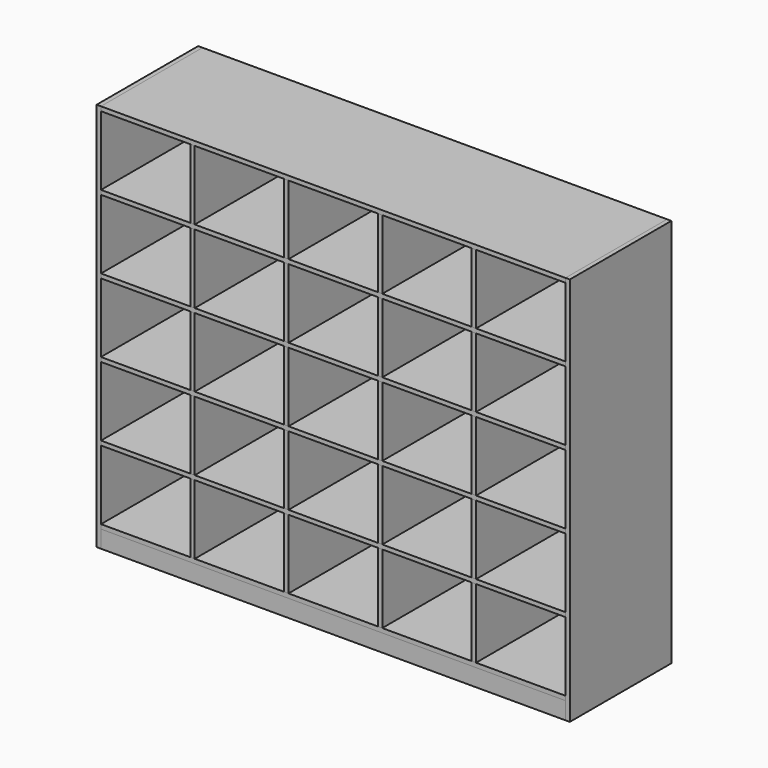
from build123d import *

# Parameters (mm, degrees)
F2_W      = 2044.7
F2_H      = 76.2
F6_DEPTH  = 19.05
F7_START  = -539.75
F7_DEPTH  = 19.05
F3_W      = 2044.7
F3_H      = 19.05
F8_DEPTH  = 558.8
F4_W      = 19.05
F4_H      = 1714.5000293255
F9_DEPTH  = 558.8
F5_W      = 19.05
F5_H      = 304.8000058651
F10_DEPTH = 558.8


# Not quite as in the source:
# - a variable given as a bare number and used for a length is read in inches; the dataset says mm whatever the document's units were


with BuildPart() as f6:
    # F2 (on Front) → F6 (new body)
    with BuildSketch(Plane.XZ):
        with Locations((0, 38.1)):
            Rectangle(F2_W, F2_H)
    extrude(amount=-F6_DEPTH)


with BuildPart() as f7:
    # F2 (on Front) → F7 (new body)
    with BuildSketch(Plane.XZ.offset(F7_START)):
        with Locations((0, 38.1)):
            Rectangle(F2_W, F2_H)
    extrude(amount=-F7_DEPTH)


with BuildPart() as f8:
    # F3 (on Front) → F8 (new body)
    with BuildSketch(Plane.XZ):
        with Locations((0, 85.725)):
            Rectangle(F3_W, F3_H)
    extrude(amount=-F8_DEPTH)


with BuildPart() as f8b:
    # F3 (on Front) → F8, piece 2 (new body)
    with BuildSketch(Plane.XZ):
        with Locations((0, 409.5750058651)):
            Rectangle(F3_W, F3_H)
    extrude(amount=-F8_DEPTH)


with BuildPart() as f8c:
    # F3 (on Front) → F8, piece 3 (new body)
    with BuildSketch(Plane.XZ):
        with Locations((0, 733.4250117302)):
            Rectangle(F3_W, F3_H)
    extrude(amount=-F8_DEPTH)


with BuildPart() as f8d:
    # F3 (on Front) → F8, piece 4 (new body)
    with BuildSketch(Plane.XZ):
        with Locations((0, 1057.2750175953)):
            Rectangle(F3_W, F3_H)
    extrude(amount=-F8_DEPTH)


with BuildPart() as f8e:
    # F3 (on Front) → F8, piece 5 (new body)
    with BuildSketch(Plane.XZ):
        with Locations((0, 1381.1250234604)):
            Rectangle(F3_W, F3_H)
    extrude(amount=-F8_DEPTH)


with BuildPart() as f8f:
    # F3 (on Front) → F8, piece 6 (new body)
    with BuildSketch(Plane.XZ):
        with Locations((0, 1704.9750293255)):
            Rectangle(F3_W, F3_H)
    extrude(amount=-F8_DEPTH)


with BuildPart() as f9:
    # F4 (on Front) → F9 (new body)
    with BuildSketch(Plane.XZ):
        with Locations((-1031.875, 857.2500146627)):
            Rectangle(F4_W, F4_H)
    extrude(amount=-F9_DEPTH)


with BuildPart() as f9b:
    # F4 (on Front) → F9, piece 2 (new body)
    with BuildSketch(Plane.XZ):
        with Locations((1031.875, 857.2500146627)):
            Rectangle(F4_W, F4_H)
    extrude(amount=-F9_DEPTH)


with BuildPart() as f10:
    # F5 (on Front) → F10 (new body)
    with BuildSketch(Plane.XZ):
        with Locations((-619.125, 247.6500029325)):
            Rectangle(F5_W, F5_H)
    extrude(amount=-F10_DEPTH)


with BuildPart() as f10b:
    # F5 (on Front) → F10, piece 2 (new body)
    with BuildSketch(Plane.XZ):
        with Locations((-619.125, 571.5000087976)):
            Rectangle(F5_W, F5_H)
    extrude(amount=-F10_DEPTH)


with BuildPart() as f10c:
    # F5 (on Front) → F10, piece 3 (new body)
    with BuildSketch(Plane.XZ):
        with Locations((-619.125, 895.3500146627)):
            Rectangle(F5_W, F5_H)
    extrude(amount=-F10_DEPTH)


with BuildPart() as f10d:
    # F5 (on Front) → F10, piece 4 (new body)
    with BuildSketch(Plane.XZ):
        with Locations((-619.125, 1219.2000205278)):
            Rectangle(F5_W, F5_H)
    extrude(amount=-F10_DEPTH)


with BuildPart() as f10e:
    # F5 (on Front) → F10, piece 5 (new body)
    with BuildSketch(Plane.XZ):
        with Locations((-619.125, 1543.0500263929)):
            Rectangle(F5_W, F5_H)
    extrude(amount=-F10_DEPTH)


with BuildPart() as f10f:
    # F5 (on Front) → F10, piece 6 (new body)
    with BuildSketch(Plane.XZ):
        with Locations((-206.374994278, 247.6500029325)):
            Rectangle(F5_W, F5_H)
    extrude(amount=-F10_DEPTH)


with BuildPart() as f10g:
    # F5 (on Front) → F10, piece 7 (new body)
    with BuildSketch(Plane.XZ):
        with Locations((-206.374994278, 571.5000087976)):
            Rectangle(F5_W, F5_H)
    extrude(amount=-F10_DEPTH)


with BuildPart() as f10h:
    # F5 (on Front) → F10, piece 8 (new body)
    with BuildSketch(Plane.XZ):
        with Locations((-206.374994278, 895.3500146627)):
            Rectangle(F5_W, F5_H)
    extrude(amount=-F10_DEPTH)


with BuildPart() as f10i:
    # F5 (on Front) → F10, piece 9 (new body)
    with BuildSketch(Plane.XZ):
        with Locations((-206.374994278, 1219.2000205278)):
            Rectangle(F5_W, F5_H)
    extrude(amount=-F10_DEPTH)


with BuildPart() as f10j:
    # F5 (on Front) → F10, piece 10 (new body)
    with BuildSketch(Plane.XZ):
        with Locations((-206.374994278, 1543.0500263929)):
            Rectangle(F5_W, F5_H)
    extrude(amount=-F10_DEPTH)


with BuildPart() as f10k:
    # F5 (on Front) → F10, piece 11 (new body)
    with BuildSketch(Plane.XZ):
        with Locations((206.3750114441, 247.6500029325)):
            Rectangle(F5_W, F5_H)
    extrude(amount=-F10_DEPTH)


with BuildPart() as f10l:
    # F5 (on Front) → F10, piece 12 (new body)
    with BuildSketch(Plane.XZ):
        with Locations((206.3750114441, 571.5000087976)):
            Rectangle(F5_W, F5_H)
    extrude(amount=-F10_DEPTH)


with BuildPart() as f10m:
    # F5 (on Front) → F10, piece 13 (new body)
    with BuildSketch(Plane.XZ):
        with Locations((206.3750114441, 895.3500146627)):
            Rectangle(F5_W, F5_H)
    extrude(amount=-F10_DEPTH)


with BuildPart() as f10n:
    # F5 (on Front) → F10, piece 14 (new body)
    with BuildSketch(Plane.XZ):
        with Locations((206.3750114441, 1219.2000205278)):
            Rectangle(F5_W, F5_H)
    extrude(amount=-F10_DEPTH)


with BuildPart() as f10o:
    # F5 (on Front) → F10, piece 15 (new body)
    with BuildSketch(Plane.XZ):
        with Locations((206.3750114441, 1543.0500263929)):
            Rectangle(F5_W, F5_H)
    extrude(amount=-F10_DEPTH)


with BuildPart() as f10p:
    # F5 (on Front) → F10, piece 16 (new body)
    with BuildSketch(Plane.XZ):
        with Locations((619.1250171661, 247.6500029325)):
            Rectangle(F5_W, F5_H)
    extrude(amount=-F10_DEPTH)


with BuildPart() as f10q:
    # F5 (on Front) → F10, piece 17 (new body)
    with BuildSketch(Plane.XZ):
        with Locations((619.1250171661, 571.5000087976)):
            Rectangle(F5_W, F5_H)
    extrude(amount=-F10_DEPTH)


with BuildPart() as f10r:
    # F5 (on Front) → F10, piece 18 (new body)
    with BuildSketch(Plane.XZ):
        with Locations((619.1250171661, 895.3500146627)):
            Rectangle(F5_W, F5_H)
    extrude(amount=-F10_DEPTH)


with BuildPart() as f10s:
    # F5 (on Front) → F10, piece 19 (new body)
    with BuildSketch(Plane.XZ):
        with Locations((619.1250171661, 1219.2000205278)):
            Rectangle(F5_W, F5_H)
    extrude(amount=-F10_DEPTH)


with BuildPart() as f10t:
    # F5 (on Front) → F10, piece 20 (new body)
    with BuildSketch(Plane.XZ):
        with Locations((619.1250171661, 1543.0500263929)):
            Rectangle(F5_W, F5_H)
    extrude(amount=-F10_DEPTH)


solid = Compound([f6.part, f7.part, f8.part, f8b.part, f8c.part, f8d.part, f8e.part, f8f.part, f9.part, f9b.part, f10.part, f10b.part, f10c.part, f10d.part, f10e.part, f10f.part, f10g.part, f10h.part, f10i.part, f10j.part, f10k.part, f10l.part, f10m.part, f10n.part, f10o.part, f10p.part, f10q.part, f10r.part, f10s.part, f10t.part])
